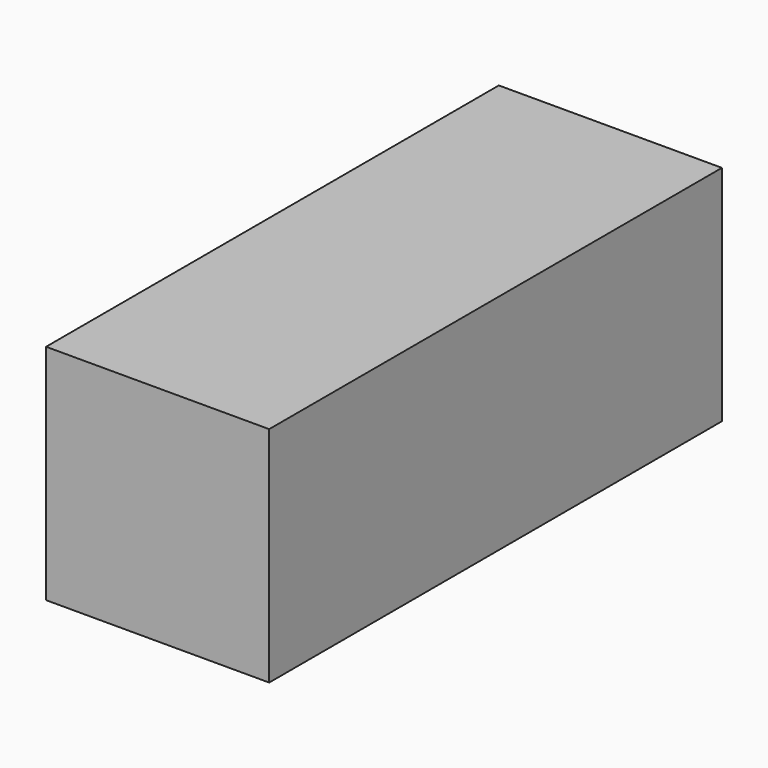
from build123d import *

# Parameters (mm, degrees)
F1_E0_BOTTOM_W = 63.4145736694
F1_E0_BOTTOM_H = 25
F2_DEPTH       = 25


with BuildPart() as f2:
    # F1_E0_bottom (on explicit) → F2 (new body)
    with BuildSketch(Plane(origin=(0, -63.4145736694, 83.9292407036), x_dir=(0, 1, 0), z_dir=(0, 0, -1))):
        with Locations((31.7072868347, 12.5)):
            Rectangle(F1_E0_BOTTOM_W, F1_E0_BOTTOM_H)
    extrude(amount=F2_DEPTH)


solid = f2.part
